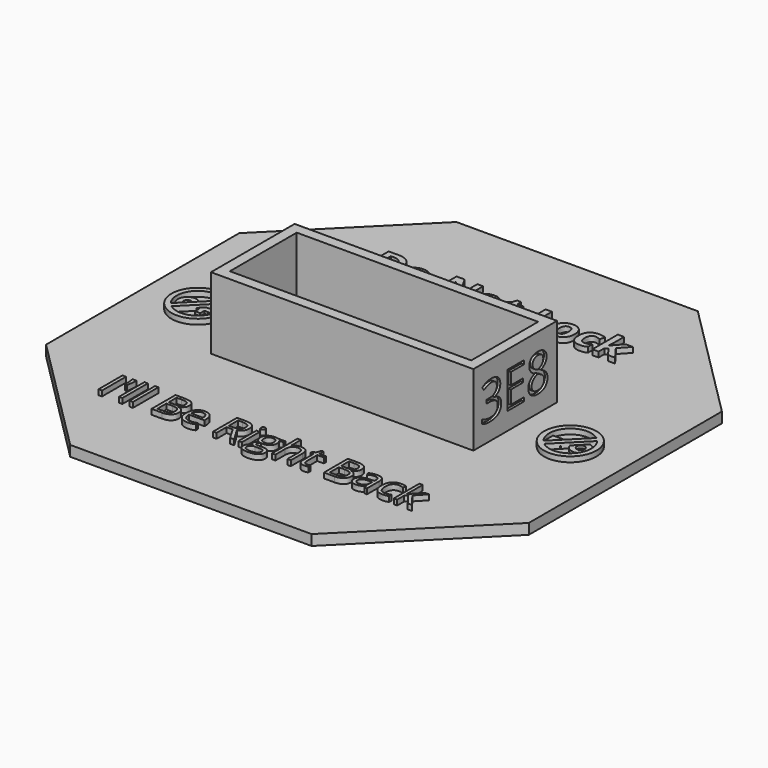
from build123d import *

# Parameters (mm, degrees)
F3_W          = 92
F3_H          = 92
F3_W_2        = 46
F3_H_2        = 15.93
F4_DEPTH      = 2
F5_W          = 50
F5_H          = 19.93
F5_W_2        = 46
F5_H_2        = 15.93
F6_DEPTH      = 13.68
F7_R          = 5
F7_TEXT_SIZE  = 7.9861111111
F8_DEPTH      = 1
F7_R_2        = 0.75
F9_DEPTH      = 0.5
F10_SIZE      = 23
F11_TEXT_SIZE = 9.7222222222
F12_DEPTH     = 0.5


# Not quite as in the source:
# - Text() gives the source's letters only with a copy of the font that has no kerning and outlines rounded to 1/6400 em; it was checked with that copy


with BuildPart() as f4:
    # F3 (on Top) → F4 (new body)
    with BuildSketch(Plane.XY):
        Rectangle(F3_W, F3_H)
        Rectangle(F3_W_2, F3_H_2, mode=Mode.SUBTRACT)
    extrude(amount=F4_DEPTH)

    # F5 (on face) → F6 (join)
    with BuildSketch(Plane.XY.offset(2)):
        Rectangle(F5_W, F5_H)
        Rectangle(F5_W_2, F5_H_2, mode=Mode.SUBTRACT)
    extrude(amount=F6_DEPTH)

    # F7 (on face) → F8 (join)
    with BuildSketch(Plane.XY.offset(2)):
        with Locations((-35.5, 0)):
            Circle(F7_R)
        with BuildLine():
            ThreePointArc((-37.9526896495, -3.1597964307), (-38.3284271247, -2.8284271247), (-38.6597964307, -2.4526896495))
            ThreePointArc((-38.6597964307, -2.4526896495), (-38.3284271247, 2.8284271247), (-33.0473103505, 3.1597964307))
            ThreePointArc((-33.0473103505, 3.1597964307), (-32.6715728753, 2.8284271247), (-32.3402035693, 2.4526896495))
            ThreePointArc((-32.3402035693, 2.4526896495), (-31.7158762096, 1.2963051873), (-31.5, 0))
            ThreePointArc((-31.5, 0), (-33.7408465954, -3.5924057815), (-37.9526896495, -3.1597964307))
        make_face(mode=Mode.SUBTRACT)
        with Locations((35.5, 0)):
            Circle(F7_R)
        with BuildLine():
            ThreePointArc((38.6597964307, 2.4526896495), (39.2841237904, 1.2963051873), (39.5, 0))
            ThreePointArc((39.5, 0), (37.2591534046, -3.5924057815), (33.0473103505, -3.1597964307))
            ThreePointArc((33.0473103505, -3.1597964307), (32.6715728753, -2.8284271247), (32.3402035693, -2.4526896495))
            ThreePointArc((32.3402035693, -2.4526896495), (32.6715728753, 2.8284271247), (37.9526896495, 3.1597964307))
            ThreePointArc((37.9526896495, 3.1597964307), (38.3284271247, 2.8284271247), (38.6597964307, 2.4526896495))
        make_face(mode=Mode.SUBTRACT)
        with Locations((-24.473063151, 25.1075)):
            Text('Do Not Lock', F7_TEXT_SIZE, font='Open Sans', font_style=FontStyle.BOLD, text_align=(TextAlign.LEFT, TextAlign.BOTTOM))
        with Locations((-30.5044487847, -30.8575)):
            Text("I'll Be Right Back", F7_TEXT_SIZE, font='Open Sans', text_align=(TextAlign.LEFT, TextAlign.BOTTOM))
        with BuildLine():
            Line((-35.7071067812, 0.5), (-34.2928932188, 0.5))
            Line((-34.2928932188, 0.5), (-32.3402035693, 2.4526896495))
            ThreePointArc((-32.3402035693, 2.4526896495), (-32.6715728753, 2.8284271247), (-33.0473103505, 3.1597964307))
            Line((-33.0473103505, 3.1597964307), (-35.7071067812, 0.5))
        make_face()
        with BuildLine():
            ThreePointArc((-35.75, 0), (-35.7683332855, -0.2526467688), (-35.8229490169, -0.5))
            Line((-35.8229490169, -0.5), (-35.2928932188, -0.5))
            Line((-35.2928932188, -0.5), (-34.2928932188, 0.5))
            Line((-34.2928932188, 0.5), (-35.7071067812, 0.5))
            Line((-35.7071067812, 0.5), (-35.79839616, 0.4087106211))
            ThreePointArc((-35.79839616, 0.4087106211), (-35.7621411565, 0.2057829926), (-35.75, 0))
        make_face()
        with BuildLine():
            ThreePointArc((-37.9087106211, -1.70160384), (-36.6264241501, -1.5163657984), (-35.8229490169, -0.5))
            ThreePointArc((-35.8229490169, -0.5), (-35.7683332855, -0.2526467688), (-35.75, 0))
            ThreePointArc((-35.75, 0), (-35.7621411565, 0.2057829926), (-35.79839616, 0.4087106211))
            Line((-35.79839616, 0.4087106211), (-37.9087106211, -1.70160384))
        make_face()
        with BuildLine():
            Line((-35.2928932188, -0.5), (-35.8229490169, -0.5))
            ThreePointArc((-35.8229490169, -0.5), (-36.6264241501, -1.5163657984), (-37.9087106211, -1.70160384))
            Line((-37.9087106211, -1.70160384), (-38.6597964307, -2.4526896495))
            ThreePointArc((-38.6597964307, -2.4526896495), (-38.3284271247, -2.8284271247), (-37.9526896495, -3.1597964307))
            Line((-37.9526896495, -3.1597964307), (-35.2928932188, -0.5))
        make_face()
        with BuildLine():
            Line((37.9087106211, 1.70160384), (38.6597964307, 2.4526896495))
            ThreePointArc((38.6597964307, 2.4526896495), (38.3284271247, 2.8284271247), (37.9526896495, 3.1597964307))
            Line((37.9526896495, 3.1597964307), (35.2928932188, 0.5))
            Line((35.2928932188, 0.5), (35.8229490169, 0.5))
            ThreePointArc((35.8229490169, 0.5), (36.6264241501, 1.5163657984), (37.9087106211, 1.70160384))
        make_face()
        with BuildLine():
            Line((35.79839616, -0.4087106211), (37.9087106211, 1.70160384))
            ThreePointArc((37.9087106211, 1.70160384), (36.6264241501, 1.5163657984), (35.8229490169, 0.5))
            ThreePointArc((35.8229490169, 0.5), (35.7506384446, 0.0472667787), (35.79839616, -0.4087106211))
        make_face()
        with BuildLine():
            Line((33.8229490169, -1.5), (34.7071067812, -1.5))
            Line((34.7071067812, -1.5), (34.8229490169, -1.3841577643))
            Line((34.8229490169, -1.3841577643), (34.8229490169, -0.5))
            Line((34.8229490169, -0.5), (35.7071067812, -0.5))
            Line((35.7071067812, -0.5), (35.79839616, -0.4087106211))
            ThreePointArc((35.79839616, -0.4087106211), (35.7506384446, 0.0472667787), (35.8229490169, 0.5))
            Line((35.8229490169, 0.5), (35.2928932188, 0.5))
            Line((35.2928932188, 0.5), (33.8229490169, -0.9699442019))
            Line((33.8229490169, -0.9699442019), (33.8229490169, -1.5))
        make_face()
        Polygon((34.8229490169, -0.5), (34.8229490169, -1.3841577643), (35.7071067812, -0.5), align=None)
        with BuildLine():
            ThreePointArc((32.3402035693, -2.4526896495), (32.6715728753, -2.8284271247), (33.0473103505, -3.1597964307))
            Line((33.0473103505, -3.1597964307), (34.7071067812, -1.5))
            Line((34.7071067812, -1.5), (33.8229490169, -1.5))
            Line((33.8229490169, -1.5), (33.8229490169, -0.9699442019))
            Line((33.8229490169, -0.9699442019), (32.3402035693, -2.4526896495))
        make_face()
    extrude(amount=F8_DEPTH)

    # F7 (on face) → F9 (join)
    with BuildSketch(Plane.XY.offset(2)):
        Polygon((-34.2928932188, 0.5), (-35.2928932188, -0.5), (-34.8229490169, -0.5), (-34.8229490169, -1.5), (-33.8229490169, -1.5), (-33.8229490169, -0.5), (-32.8229490169, -0.5), (-32.8229490169, -1.5), (-31.8229490169, -1.5), (-31.8229490169, 0.5), align=None)
        with BuildLine():
            ThreePointArc((-35.8229490169, 0.5), (-38.7704080783, 1.2035627589), (-37.9087106211, -1.70160384))
            Line((-37.9087106211, -1.70160384), (-35.79839616, 0.4087106211))
            ThreePointArc((-35.79839616, 0.4087106211), (-35.8100560539, 0.4545211315), (-35.8229490169, 0.5))
        make_face()
        with Locations((-37.5, 0)):
            Circle(F7_R_2, mode=Mode.SUBTRACT)
        with BuildLine():
            ThreePointArc((39.25, 0), (38.8743623225, 1.0833412235), (37.9087106211, 1.70160384))
            Line((37.9087106211, 1.70160384), (35.79839616, -0.4087106211))
            ThreePointArc((35.79839616, -0.4087106211), (35.8100560539, -0.4545211315), (35.8229490169, -0.5))
            ThreePointArc((35.8229490169, -0.5), (37.7526467688, -1.7316667145), (39.25, 0))
        make_face()
        with Locations((37.5, 0)):
            Circle(F7_R_2, mode=Mode.SUBTRACT)
        Polygon((33.8229490169, -0.9699442019), (35.2928932188, 0.5), (31.8229490169, 0.5), (31.8229490169, -1.5), (32.8229490169, -1.5), (32.8229490169, -0.5), (33.8229490169, -0.5), align=None)
        Polygon((34.8229490169, -1.3841577643), (34.7071067812, -1.5), (34.8229490169, -1.5), align=None)
    extrude(amount=F9_DEPTH)

    # F10
    f10_edges = [f4.edges().sort_by_distance(p)[0] for p in [
        (-46, 46, 1),
        (-46, -46, 1),
        (46, -46, 1),
        (46, 46, 1),
    ]]
    chamfer(f10_edges, length=F10_SIZE)

    # F11 (on face) → F12 (cut)
    with BuildSketch(Plane.YZ.offset(25)):
        with Locations((-8.3254123264, 5.34)):
            Text('3E8', F11_TEXT_SIZE, font='Open Sans', text_align=(TextAlign.LEFT, TextAlign.BOTTOM))
    extrude(amount=-F12_DEPTH, mode=Mode.SUBTRACT)


solid = f4.part
